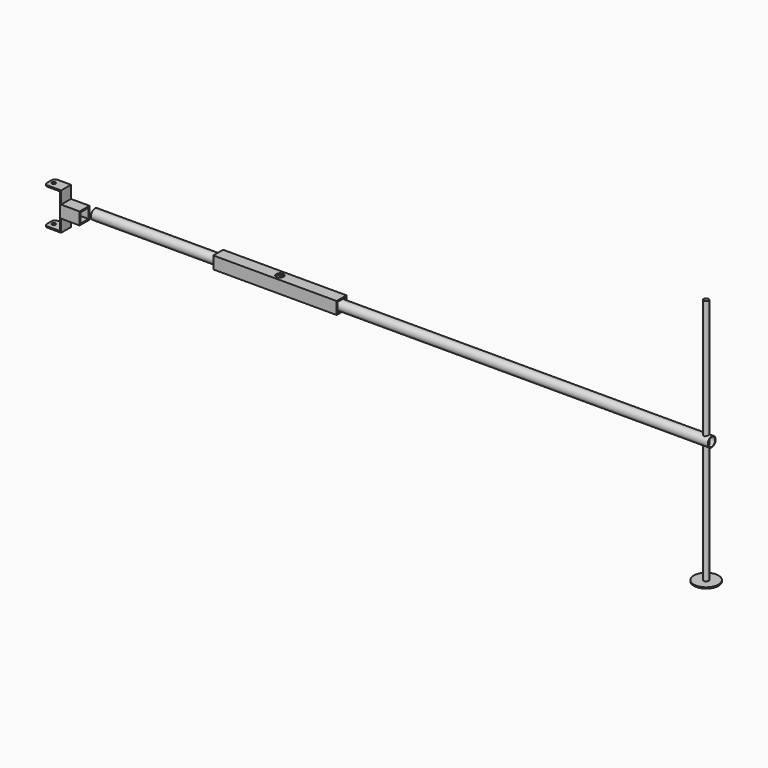
from build123d import *

# Parameters (mm, degrees)
F0_W          = 20
F0_H          = 20
F0_W_2        = 16
F0_H_2        = 16
F1_DEPTH      = 200
F2_R          = 8
F2_R_2        = 7
F3_DEPTH      = 800
F3_DEPTH_BACK = 200
F4_R          = 6
F5_DEPTH      = 25
F6_R          = 4
F7_DEPTH      = 12.5
F8_DEPTH      = 200
F9_T          = -0.5
F10_R         = 20
F11_DEPTH     = 2
F13_DEPTH     = 20
F14_T         = -2
F15_R         = 3
F16_DEPTH     = 231.2414921874
F17_R         = 5


with BuildPart() as f1:
    # F0 (on Right) → F1 (new body)
    with BuildSketch(Plane.YZ):
        Rectangle(F0_W, F0_H)
        Rectangle(F0_W_2, F0_H_2, mode=Mode.SUBTRACT)
    extrude(amount=F1_DEPTH)

    # F4 (on face) → F5 (cut)
    with BuildSketch(Plane(origin=(0, 0, -10), x_dir=(1, 0, 0), z_dir=(0, 0, -1))):
        with Locations((100, 0)):
            Circle(F4_R)
    extrude(amount=-F5_DEPTH, mode=Mode.SUBTRACT)


with BuildPart() as f3:
    # F2 (on Right) → F3 (new body, two sides)
    with BuildSketch(Plane.YZ) as f3_sk:
        Circle(F2_R)
        Circle(F2_R_2, mode=Mode.SUBTRACT)
    extrude(amount=F3_DEPTH)
    extrude(f3_sk.sketch, amount=-F3_DEPTH_BACK)

    # F6 (on Top) → F7 (cut, symmetric)
    with BuildSketch(Plane.XY):
        with Locations((791, 0)):
            Circle(F6_R)
    extrude(amount=F7_DEPTH, both=True, mode=Mode.SUBTRACT)


with BuildPart() as f8:
    # F6 (on Top) → F8 (new body, symmetric)
    with BuildSketch(Plane.XY):
        with Locations((791, 0)):
            Circle(F6_R)
    extrude(amount=F8_DEPTH, both=True)

    # F9
    f9_openings = [f8.faces().sort_by_distance(p)[0] for p in [
        (791, 0, 200),
        (791, 0, -200),
    ]]
    offset(amount=F9_T, openings=f9_openings)


with BuildPart() as f11:
    # F10 (on face) → F11 (new body)
    with BuildSketch(Plane(origin=(0, 0, -200), x_dir=(1, 0, 0), z_dir=(0, 0, -1))):
        with Locations((791, 0)):
            Circle(F10_R)
    extrude(amount=F11_DEPTH)


with BuildPart() as f13:
    # F12 (on Front) → F13 (new body)
    with BuildSketch(Plane.XZ):
        Polygon((-238.6837440729, -11.0095078126), (-208.6837440729, -11.0095078126), (-208.6837440729, 8.9904921874), (-238.6837440729, 8.9904921874), (-238.6837440729, 29.2404921874), (-265.6837440729, 29.2404921874), (-265.6837440729, 27.2404921874), (-240.6837440729, 27.2404921874), (-240.6837440729, -29.2595078126), (-265.6837440729, -29.2595078126), (-265.6837440729, -31.2595078126), (-238.6837440729, -31.2595078126), align=None)
    extrude(amount=F13_DEPTH)

    # F14
    f14_openings = [f13.faces().sort_by_distance(p)[0] for p in [
        (-208.683744, -10, -1.009508),
    ]]
    offset(amount=F14_T, openings=f14_openings, kind=Kind.INTERSECTION)

    # F15 (on face) → F16 (cut, through all)
    with BuildSketch(Plane.XY.offset(29.2404921874)):
        with Locations((-258.6837440729, -10)):
            Circle(F15_R)
    extrude(amount=-F16_DEPTH, mode=Mode.SUBTRACT)

    # F17
    f17_edges = [f13.edges().sort_by_distance(p)[0] for p in [
        (-265.683744, -20, 28.240492),
        (-265.683744, 0, 28.240492),
        (-265.683744, -20, -30.259508),
        (-265.683744, 0, -30.259508),
    ]]
    fillet(f17_edges, radius=F17_R)


solid = Compound([f1.part, f3.part, f8.part, f11.part, f13.part])
